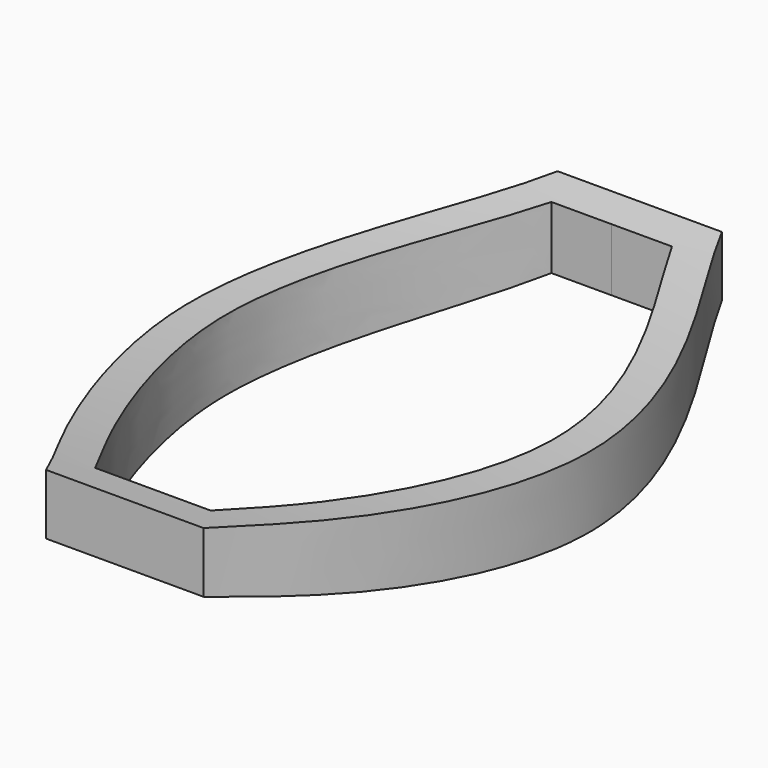
from build123d import *

# Parameters (mm, degrees)
F1_DEPTH = 17.78
F4_START = 50.8
F4_DEPTH = 101.6


# Not quite as in the source:
# - ends of sketch curves that miss each other by under 0.0002 mm in the source are joined
# - the dataset's text gives a spline's control points without its knots; the knots are read off the source's solid


with BuildPart() as f1:
    # F0 (on Top) → F1 (new body)
    with BuildSketch(Plane.XY):
        with BuildLine():
            add(Edge.make_bspline(
                [(-14.2528750466, -58.1654505452), (-16.7148857825, -53.2837046852), (-24.6397666055, -41.5790941252), (-42.0443551665, 0.28539923), (-27.9347681105, 36.4149676999), (-18.0333241185, 51.476303251), (-14.8739422643, 58.3434208904)],
                knots=[0, 0, 0, 0, 0.1974649281, 0.4960845553, 0.7740593431, 1, 1, 1, 1], degree=3))
            Line((-14.2528750466, -58.1654505452), (0, -58.1654505452))
            Line((0, -58.1654505452), (0, -51.8154505452))
            Line((0, -51.8154505452), (-10.4527839192, -51.8154505452))
            add(Edge.make_bspline(
                [(-10.4527839192, -51.8154505452), (-10.728771505, -51.3241731046), (-11.939437541, -49.2032153167), (-13.6932783853, -46.2483150477), (-15.7536448938, -42.6416240641), (-17.0939529837, -40.189108658), (-18.2006251765, -38.0697762193), (-19.3305409812, -35.8348768336), (-20.7684428163, -32.8448146104), (-22.4835161729, -28.9935186051), (-24.688286119, -23.5781743742), (-26.6687214464, -17.8482408642), (-28.2295627767, -12.0251421867), (-28.9921200238, -8.3956407392), (-29.453064017, -5.527756516), (-29.7193606137, -3.4028772539), (-29.9019099727, -1.3096576507), (-29.9960045187, 0.7365518632), (-30.0009841043, 2.7630533504), (-29.8956963568, 5.4471848741), (-29.5639281326, 8.7649348477), (-28.8781885559, 12.6836208634), (-27.6244181361, 17.8143414607), (-25.9293365538, 22.7839852238), (-23.9389531615, 27.5449593825), (-22.3369239237, 30.9996677952), (-20.6654192015, 34.3255629483), (-18.9603824943, 37.518870095), (-17.2379027842, 40.6135304724), (-14.943864558, 44.6477066774), (-12.8096121303, 48.3999683751), (-11.3253177791, 51.1951563129), (-10.9136410124, 51.9933721491)],
                knots=[0.0437399964, 0.0437399964, 0.0437399964, 0.0437399964, 0.0625, 0.125, 0.15625, 0.1875, 0.203125, 0.21875, 0.25, 0.28125, 0.3125, 0.375, 0.40625, 0.4375, 0.453125, 0.46875, 0.484375, 0.5, 0.515625, 0.53125, 0.5625, 0.59375, 0.625, 0.6875, 0.71875, 0.75, 0.78125, 0.8125, 0.84375, 0.875, 0.9375, 0.962256316, 0.962256316, 0.962256316, 0.962256316], degree=3))
            Line((-10.9136410124, 51.9933721491), (0, 51.9934208904))
            Line((0, 51.9934208904), (0, 58.3434208904))
            Line((0, 58.3434208904), (-14.8739422643, 58.3434208904))
        make_face()
    extrude(amount=F1_DEPTH)

    # F2: F1 across plane


with BuildPart() as f1_1:
    add(f1.part)
    add(f1.part.mirror(Plane.YZ))

    # F3 (on Right) → F4 (intersect)
    with BuildSketch(Plane.YZ.offset(F4_START)):
        with BuildLine():
            ThreePointArc((140.51924313, 42.7512294533), (0, 12.8061219354), (-140.51924313, 42.7512294533))
            ThreePointArc((-140.51924313, 42.7512294533), (0, 0), (140.51924313, 42.7512294533))
        make_face()
    extrude(amount=-F4_DEPTH, mode=Mode.INTERSECT)


solid = f1_1.part
